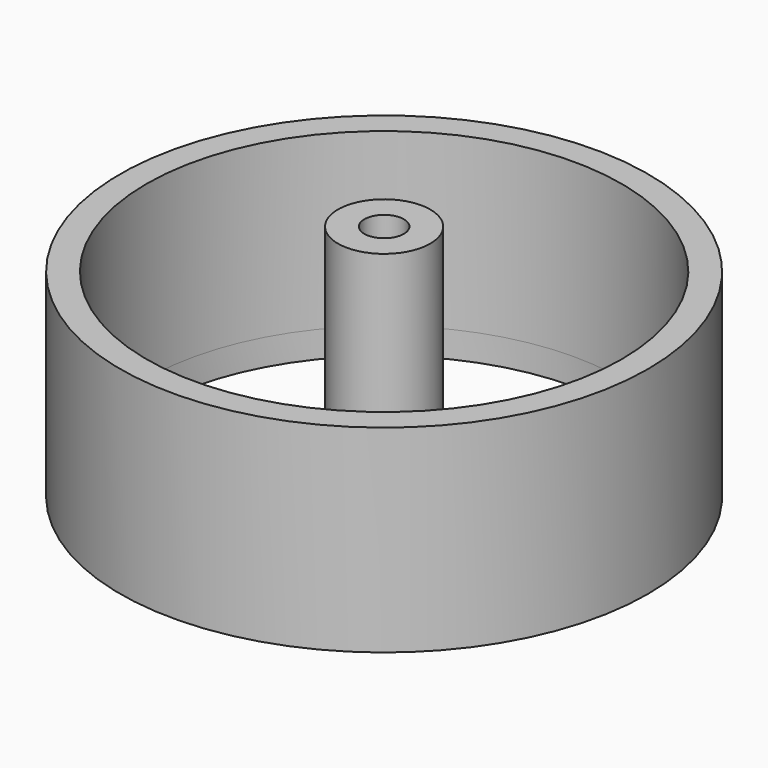
from build123d import *

# Parameters (mm, degrees)
F0_R      = 20
F1_DEPTH  = 15
F2_R      = 18
F3_DEPTH  = 13
F4_R      = 3.5
F4_R_2    = 1.5
F5_DEPTH  = 13
F6_R      = 3.5
F6_R_2    = 1.5
F7_DEPTH  = 3
F10_DEPTH = 2


with BuildPart() as f1:
    # F0 (on Top) → F1 (new body)
    with BuildSketch(Plane.XY):
        Circle(F0_R)
    extrude(amount=F1_DEPTH)

    # F2 (on face) → F3 (cut)
    with BuildSketch(Plane.XY.offset(15)):
        Circle(F2_R)
    extrude(amount=-F3_DEPTH, mode=Mode.SUBTRACT)

    # F4 (on face) → F5 (join)
    with BuildSketch(Plane.XY.offset(15)):
        Circle(F4_R)
        Circle(F4_R_2, mode=Mode.SUBTRACT)
    extrude(amount=-F5_DEPTH)

    # F6 (on face) → F7 (join)
    with BuildSketch(Plane.XY.offset(15)):
        Circle(F6_R)
        Circle(F6_R_2, mode=Mode.SUBTRACT)
    extrude(amount=F7_DEPTH)

    # F9 (on face) → F10 (cut)
    with BuildSketch(Plane(origin=(0, 0, 0), x_dir=(1, 0, 0), z_dir=(0, 0, -1))):
        with BuildLine():
            Line((-2.9190978863, 4.0177935548), (-1.6146279111, 17.9274364232))
            ThreePointArc((-1.6146279111, 17.9274364232), (-10.5801345413, 14.5623058987), (-16.5510577667, 7.0754849166))
            Line((-16.5510577667, 7.0754849166), (-2.9190978863, 4.0177935548))
        make_face()
        with BuildLine():
            ThreePointArc((-17.5489526949, 4.0042801241), (-17.1190172933, -5.5623058987), (-11.8437441606, -13.5545462579))
            Line((-11.8437441606, -13.5545462579), (-4.7231995965, -1.5346605781))
            Line((-4.7231995965, -1.5346605781), (-17.5489526949, 4.0042801241))
        make_face()
        with BuildLine():
            ThreePointArc((-9.2312213213, -15.452655206), (0, -18), (9.2312213213, -15.452655206))
            Line((9.2312213213, -15.452655206), (0, -4.9662659533))
            Line((0, -4.9662659533), (-9.2312213213, -15.452655206))
        make_face()
        with BuildLine():
            ThreePointArc((11.8437441606, -13.5545462579), (16.3888284342, -7.4435409957), (18, 0))
            ThreePointArc((18, 0), (17.8868827428, 2.0148016642), (17.5489526949, 4.0042801241))
            Line((17.5489526949, 4.0042801241), (4.7231995965, -1.5346605781))
            Line((4.7231995965, -1.5346605781), (11.8437441606, -13.5545462579))
        make_face()
        with BuildLine():
            Line((2.9190978863, 4.0177935548), (16.5510577667, 7.0754849166))
            ThreePointArc((16.5510577667, 7.0754849166), (10.5801345413, 14.5623058987), (1.6146279111, 17.9274364232))
            Line((1.6146279111, 17.9274364232), (2.9190978863, 4.0177935548))
        make_face()
        with BuildLine():
            Line((-1.3322676027, -3.4528501024), (-1.6587573928, -3.0819675391))
            ThreePointArc((-1.6587573928, -3.0819675391), (-2.057248383, -2.8315594803), (-2.4185410871, -2.5299523731))
            Line((-2.4185410871, -2.5299523731), (-2.8721622593, -2.3340511457))
            Line((-2.8721622593, -2.3340511457), (-8.0671256706, -11.1034459232))
            Line((-8.0671256706, -11.1034459232), (-1.3322676027, -3.4528501024))
        make_face()
        with BuildLine():
            Line((2.8721622593, -2.3340511457), (2.4185410871, -2.5299523731))
            ThreePointArc((2.4185410871, -2.5299523731), (2.057248383, -2.8315594803), (1.6587573928, -3.0819675391))
            Line((1.6587573928, -3.0819675391), (1.3322676027, -3.4528501024))
            Line((1.3322676027, -3.4528501024), (8.0671256706, -11.1034459232))
            Line((8.0671256706, -11.1034459232), (2.8721622593, -2.3340511457))
        make_face()
        with BuildLine():
            ThreePointArc((3.1534979878, 1.5183709826), (3.328697807, 1.0815594803), (3.443709535, 0.6251916817))
            Line((3.443709535, 0.6251916817), (3.6955489199, 0.2000724244))
            Line((3.6955489199, 0.2000724244), (13.0528835265, 4.2411389504))
            Line((13.0528835265, 4.2411389504), (3.1073615002, 2.0103271628))
            Line((3.1073615002, 2.0103271628), (3.1534979878, 1.5183709826))
        make_face()
        with BuildLine():
            ThreePointArc((-0.4695721472, 3.4683572478), (0, 3.5), (0.4695721472, 3.4683572478))
            Line((0.4695721472, 3.4683572478), (0.9517072369, 3.5765016608))
            Line((0.9517072369, 3.5765016608), (0, 13.7246139455))
            Line((0, 13.7246139455), (-0.9517072369, 3.5765016608))
            Line((-0.9517072369, 3.5765016608), (-0.4695721472, 3.4683572478))
        make_face()
        with BuildLine():
            ThreePointArc((-3.443709535, 0.6251916817), (-3.328697807, 1.0815594803), (-3.1534979878, 1.5183709826))
            Line((-3.1534979878, 1.5183709826), (-3.1073615002, 2.0103271628))
            Line((-3.1073615002, 2.0103271628), (-13.0528835265, 4.2411389504))
            Line((-13.0528835265, 4.2411389504), (-3.6955489199, 0.2000724244))
            Line((-3.6955489199, 0.2000724244), (-3.443709535, 0.6251916817))
        make_face()
    extrude(amount=-F10_DEPTH, mode=Mode.SUBTRACT)


solid = f1.part
